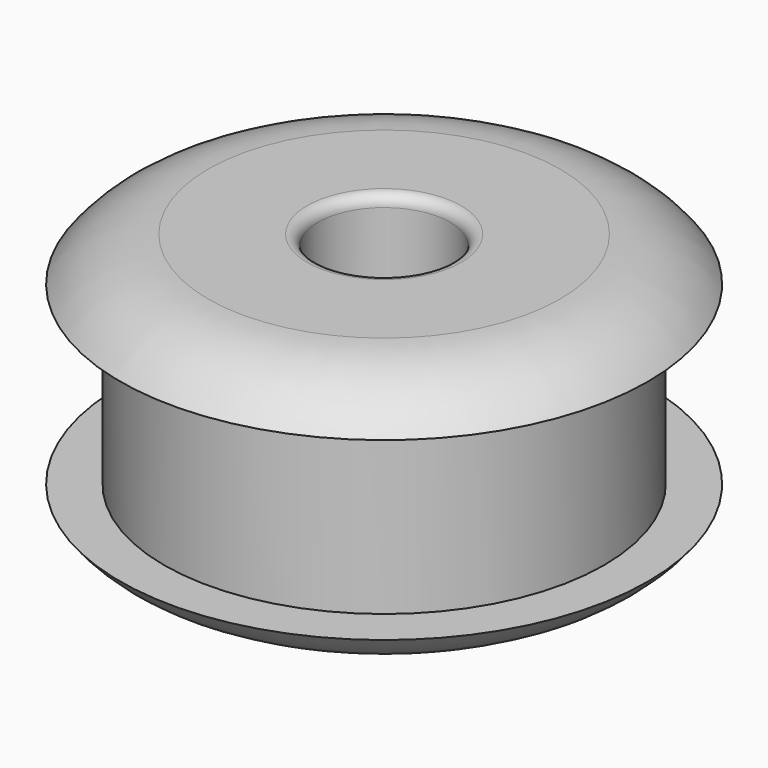
from build123d import *

# Parameters (mm, degrees)
F0_R      = 10
F1_DEPTH  = 8
F2_R      = 12
F2_R_2    = 10
F3_DEPTH  = 2
F4_R      = 12
F4_R_2    = 10
F5_DEPTH  = 2
F6_R      = 3
F7_DEPTH  = 25
F9_R      = 5
F9_R_2    = 3
F10_DEPTH = 1
F11_R     = 0.5
F13_R     = 0.5


# Not quite as in the source:
# - a fillet or chamfer that OpenCascade refuses, or shapes differently, is made with other operations: its cross-section is extruded or revolved along the edge and cut away or added


with BuildPart() as f1:
    # F0 (on Top) → F1 (new body)
    with BuildSketch(Plane.XY):
        Circle(F0_R)
    extrude(amount=F1_DEPTH)

    # F2 (on face) → F3 (join)
    with BuildSketch(Plane.XY.offset(8)):
        Circle(F2_R)
        Circle(F2_R_2, mode=Mode.SUBTRACT)
        Circle(F2_R_2)
    extrude(amount=F3_DEPTH)

    # F4 (on face) → F5 (join)
    with BuildSketch(Plane(origin=(0, 0, 0), x_dir=(1, 0, 0), z_dir=(0, 0, -1))):
        Circle(F4_R)
        Circle(F4_R_2, mode=Mode.SUBTRACT)
        Circle(F4_R_2)
    extrude(amount=F5_DEPTH)

    # F6 (on face) → F7 (cut)
    with BuildSketch(Plane(origin=(0, 0, -2), x_dir=(1, 0, 0), z_dir=(0, 0, -1))):
        Circle(F6_R)
    extrude(amount=-F7_DEPTH, mode=Mode.SUBTRACT)

    # F8: union 

    # F9 (on face) → F10 (join)
    with BuildSketch(Plane(origin=(0, 0, -2), x_dir=(1, 0, 0), z_dir=(0, 0, -1))):
        Circle(F9_R)
        Circle(F9_R_2, mode=Mode.SUBTRACT)
    extrude(amount=F10_DEPTH)

    # F11
    f11_edges = [f1.edges().sort_by_distance(p)[0] for p in [
        (-3, 0, -3),
    ]]
    fillet(f11_edges, radius=F11_R)

    # F12: fillet of radius 5 on 2 edges, made by hand

    # F12_s1 → F12_t2 (revolve, cut)
    with BuildSketch(Plane.XZ):
        with BuildLine():
            ThreePointArc((8, -2), (10.2360679775, -1.472135955), (12, 0))
            Line((12, 0), (12, -2))
            Line((12, -2), (8, -2))
        make_face()
    revolve(axis=Axis((0, 0, -2), (0, 0, -1)), mode=Mode.SUBTRACT)

    # F12_s3 → F12_t4 (revolve, cut)
    with BuildSketch(Plane.XZ):
        with BuildLine():
            ThreePointArc((8, 10), (10.2360679775, 9.472135955), (12, 8))
            Line((12, 8), (12, 10))
            Line((12, 10), (8, 10))
        make_face()
    revolve(axis=Axis((0, 0, 10), (0, 0, 1)), mode=Mode.SUBTRACT)

    # F13
    f13_edges = [f1.edges().sort_by_distance(p)[0] for p in [
        (3, 0, 4),
        (-3, 0, 10),
        (-3, 0, -2),
        (3, 0, -2.25),
        (-3, 0, -2.5),
    ]]
    fillet(f13_edges, radius=F13_R)


solid = f1.part
